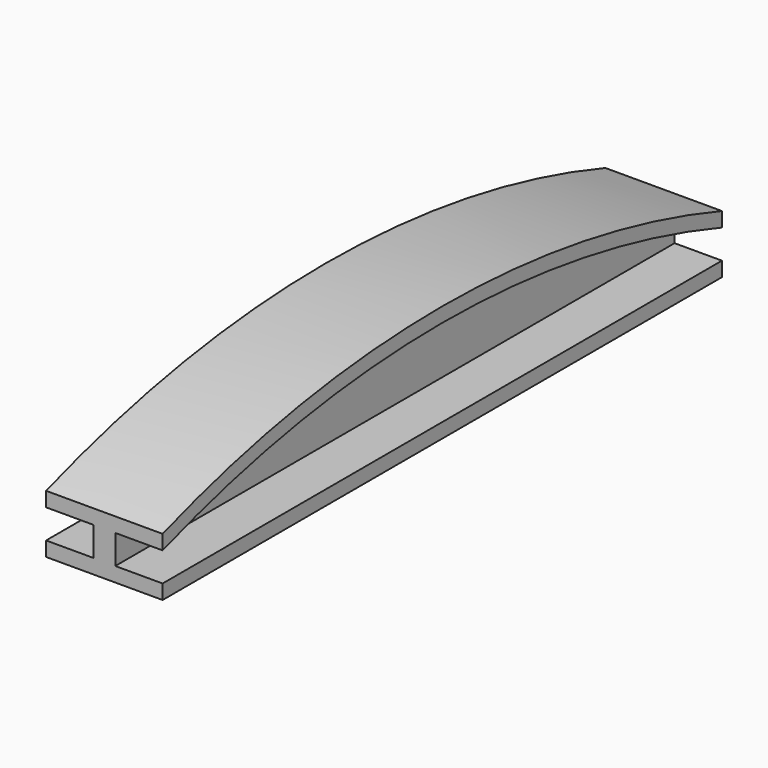
from build123d import *

# Parameters (mm, degrees)
F0_W     = 304.8
F0_H     = 6.35
F1_DEPTH = 50.8
F3_DEPTH = 0.8125
F5_DEPTH = 20.6502


# Not quite as in the source:
# - a pattern or mirror of a feature is missing from the dataset's text; its kind, count and spacing are read off the source's solid


with BuildPart() as f1:
    # F0 (on Right) → F1 (new body)
    with BuildSketch(Plane.YZ):
        with BuildLine():
            Line((-304.8, 6.35), (0, 6.35))
            Line((0, 6.35), (0, 19.05))
            ThreePointArc((0, 19.05), (-152.4, 44.45), (-304.8, 19.05))
            Line((-304.8, 19.05), (-304.8, 6.35))
        make_face()
        with BuildLine():
            ThreePointArc((-304.8, 19.05), (-152.4, 44.45), (0, 19.05))
            Line((0, 19.05), (0, 25.4))
            ThreePointArc((0, 25.4), (-152.4, 50.8), (-304.8, 25.4))
            Line((-304.8, 25.4), (-304.8, 19.05))
        make_face()
        with Locations((-152.4, 3.175)):
            Rectangle(F0_W, F0_H)
    extrude(amount=F1_DEPTH)

    # F2 (on face) → F3 (cut)
    with BuildSketch(Plane.YZ.offset(50.8)):
        with BuildLine():
            Line((0, 6.35), (0, 19.05))
            ThreePointArc((0, 19.05), (-152.4, 44.45), (-304.8, 19.05))
            Line((-304.8, 19.05), (-304.8, 6.35))
            Line((-304.8, 6.35), (0, 6.35))
        make_face()
    extrude(amount=-F3_DEPTH, mode=Mode.SUBTRACT)

    # F4 (on face) → F5 (cut)
    with BuildSketch(Plane(origin=(0, 0, 0), x_dir=(0, -1, 0), z_dir=(-1, 0, 0))):
        with BuildLine():
            Line((304.8, 6.35), (304.8, 19.05))
            ThreePointArc((304.8, 19.05), (152.4, 44.45), (0, 19.05))
            Line((0, 19.05), (0, 6.35))
            Line((0, 6.35), (304.8, 6.35))
        make_face()
    f5 = extrude(amount=-F5_DEPTH, mode=Mode.SUBTRACT)

    # F5_copies: F5 across plane
    add(f5.mirror(Plane(origin=(25.40635, 0, 0), x_dir=(0, 0, 1), z_dir=(1, 0, 0))), mode=Mode.SUBTRACT)


solid = f1.part
